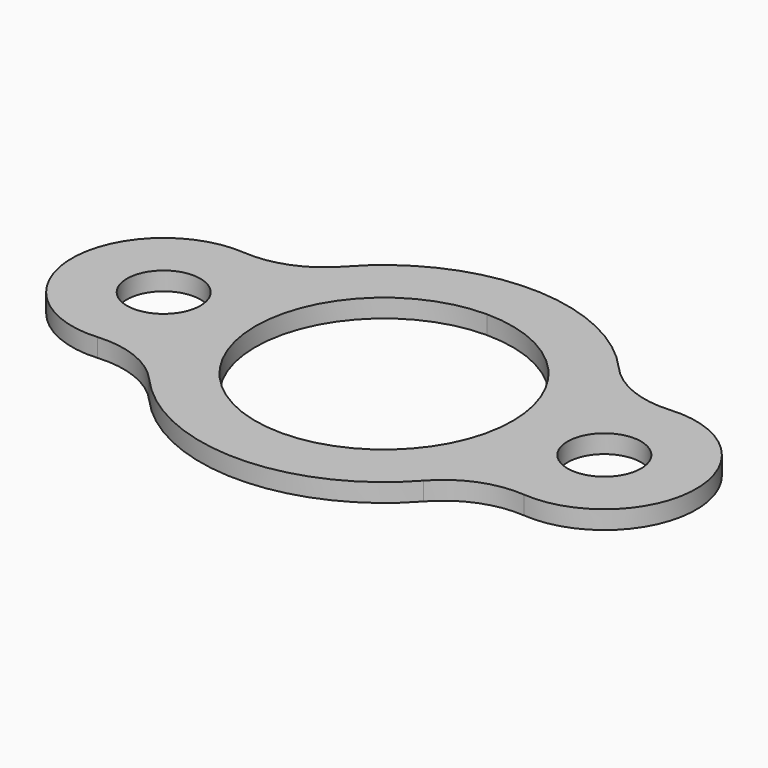
from build123d import *

# Parameters (mm, degrees)
F0_R     = 12.7
F1_DEPTH = 6.35


# Not quite as in the source:
# - a length typed as a fraction of an inch, garbled in the dataset ("3 / 203.2 mm" for 3/8 in), is restored


with BuildPart() as f1:
    # F0 (on Top) → F1 (new body)
    with BuildSketch(Plane.XY):
        with BuildLine():
            ThreePointArc((-73.6864583333, -31.6503492602), (-59.3280711503, -33.8428959089), (-47.4486111111, -42.2004656802))
            ThreePointArc((-47.4486111111, -42.2004656802), (0, -63.5), (47.4486111111, -42.2004656802))
            ThreePointArc((47.4486111111, -42.2004656802), (59.3280711503, -33.8428959089), (73.6864583333, -31.6503492602))
            ThreePointArc((73.6864583333, -31.6503492602), (107.95, 0), (73.6864583333, 31.6503492602))
            ThreePointArc((73.6864583333, 31.6503492602), (59.3280711503, 33.8428959089), (47.4486111111, 42.2004656802))
            ThreePointArc((47.4486111111, 42.2004656802), (0, 63.5), (-47.4486111111, 42.2004656802))
            ThreePointArc((-47.4486111111, 42.2004656802), (-59.3280711503, 33.8428959089), (-73.6864583333, 31.6503492602))
            ThreePointArc((-73.6864583333, 31.6503492602), (-107.95, 0), (-73.6864583333, -31.6503492602))
        make_face()
        with Locations((-76.2, 0)):
            Circle(F0_R, mode=Mode.SUBTRACT)
        with BuildLine():
            ThreePointArc((0, 44.45), (31.4308964237, 31.4308964237), (44.45, 0))
            ThreePointArc((44.45, 0), (31.4308964237, -31.4308964237), (0, -44.45))
            ThreePointArc((0, -44.45), (-44.45, 0), (0, 44.45))
        make_face(mode=Mode.SUBTRACT)
        with Locations((76.2, 0)):
            Circle(F0_R, mode=Mode.SUBTRACT)
    extrude(amount=F1_DEPTH)


solid = f1.part
